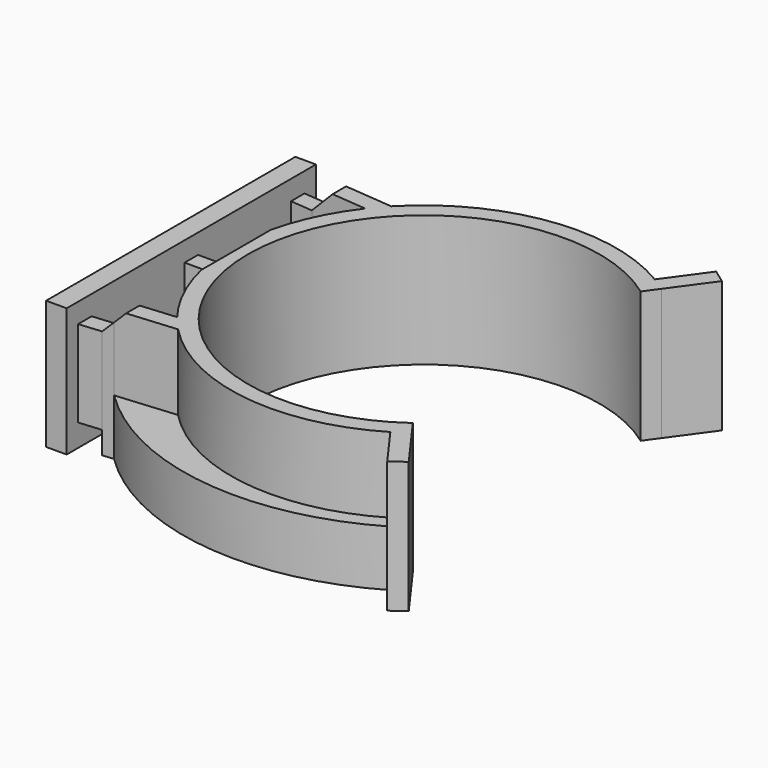
from build123d import *

# Parameters (mm, degrees)
F1_DEPTH = 11.74
F2_DEPTH = 5
F3_START = 2
F0_W     = 2
F0_H     = 1.5
F3_DEPTH = 7.74
F4_START = 2
F4_DEPTH = 3
F5_SIZE  = 2
F6_DEPTH = 11.5


# Not quite as in the source:
# - a feature names something its author has since deleted; it is built from what else it names


with BuildPart() as f1:
    # F0 (on Top) → F1 (new body)
    with BuildSketch(Plane.XY):
        with BuildLine():
            Line((5.4135556037, 0.75), (3.84, 0.75))
            Line((3.84, 0.75), (3.84, -0.75))
            Line((3.84, -0.75), (5.4135556037, -0.75))
            ThreePointArc((5.4135556037, -0.75), (5.3971960795, 0), (5.4135556037, 0.75))
        make_face()
        with BuildLine():
            ThreePointArc((10.1768930953, 11.8985744432), (9.5563193063, 11.2149691478), (8.9733212638, 10.499049243))
            ThreePointArc((8.9733212638, 10.499049243), (6.4405646269, 5.8994287949), (5.4135556037, 0.75))
            ThreePointArc((5.4135556037, 0.75), (5.3971960795, 0), (5.4135556037, -0.75))
            ThreePointArc((5.4135556037, -0.75), (6.4405646269, -5.8994287949), (8.9733212638, -10.499049243))
            ThreePointArc((8.9733212638, -10.499049243), (9.5563193063, -11.2149691478), (10.1768930953, -11.8985744432))
            ThreePointArc((10.1768930953, -11.8985744432), (20.3005620248, -17.0459811105), (31.425549646, -14.7614421147))
            ThreePointArc((31.425549646, -14.7614421147), (32.0614181574, -14.3620507052), (32.6792487822, -13.9352866242))
            Line((32.6792487822, -13.9352866242), (31.8, -12.72))
            ThreePointArc((31.8, -12.72), (6.8971960795, 0), (31.8, 12.72))
            Line((31.8, 12.72), (32.6792487822, 13.9352866242))
            ThreePointArc((32.6792487822, 13.9352866242), (32.0614181574, 14.3620507052), (31.425549646, 14.7614421147))
            ThreePointArc((31.425549646, 14.7614421147), (20.3005620248, 17.0459811105), (10.1768930953, 11.8985744432))
        make_face()
        with BuildLine():
            Line((31.425549646, -14.7614421147), (32.2020357723, -15.8346914866))
            Line((32.2020357723, -15.8346914866), (34.0313686021, -18.3631723491))
            Line((34.0313686021, -18.3631723491), (35.2466552263, -17.4839235669))
            Line((35.2466552263, -17.4839235669), (32.6792487822, -13.9352866242))
            ThreePointArc((32.6792487822, -13.9352866242), (32.0614181574, -14.3620507052), (31.425549646, -14.7614421147))
        make_face()
        with BuildLine():
            Line((34.0313686021, 18.3631723491), (32.2020357723, 15.8346914866))
            Line((32.2020357723, 15.8346914866), (31.425549646, 14.7614421147))
            ThreePointArc((31.425549646, 14.7614421147), (32.0614181574, 14.3620507052), (32.6792487822, 13.9352866242))
            Line((32.6792487822, 13.9352866242), (35.2466552263, 17.4839235669))
            Line((35.2466552263, 17.4839235669), (34.0313686021, 18.3631723491))
        make_face()
        with BuildLine():
            Line((4.84, 12.37), (3.84, 12.4583333333))
            Line((3.84, 12.4583333333), (3.84, 10.9524926213))
            Line((3.84, 10.9524926213), (8.9733212638, 10.499049243))
            ThreePointArc((8.9733212638, 10.499049243), (9.5563193063, 11.2149691478), (10.1768930953, 11.8985744432))
            Line((10.1768930953, 11.8985744432), (4.84, 12.37))
        make_face()
        with BuildLine():
            Line((3.84, -10.9524926213), (3.84, -12.4583333333))
            Line((3.84, -12.4583333333), (4.84, -12.37))
            Line((4.84, -12.37), (10.1768930953, -11.8985744432))
            ThreePointArc((10.1768930953, -11.8985744432), (9.5563193063, -11.2149691478), (8.9733212638, -10.499049243))
            Line((8.9733212638, -10.499049243), (3.84, -10.9524926213))
        make_face()
    extrude(amount=F1_DEPTH)

    # F0 (on Top) → F2 (join)
    with BuildSketch(Plane.XY):
        with BuildLine():
            ThreePointArc((32.2020357723, 15.8346914866), (17.9343865068, 18.7352052196), (4.84, 12.37))
            Line((4.84, 12.37), (10.1768930953, 11.8985744432))
            ThreePointArc((10.1768930953, 11.8985744432), (20.3005620248, 17.0459811105), (31.425549646, 14.7614421147))
            Line((31.425549646, 14.7614421147), (32.2020357723, 15.8346914866))
        make_face()
        with BuildLine():
            Line((10.1768930953, -11.8985744432), (4.84, -12.37))
            ThreePointArc((4.84, -12.37), (17.9343865068, -18.7352052196), (32.2020357723, -15.8346914866))
            Line((32.2020357723, -15.8346914866), (31.425549646, -14.7614421147))
            ThreePointArc((31.425549646, -14.7614421147), (20.3005620248, -17.0459811105), (10.1768930953, -11.8985744432))
        make_face()
        with BuildLine():
            Line((3.84, -0.75), (3.84, -10.9524926213))
            Line((3.84, -10.9524926213), (8.9733212638, -10.499049243))
            ThreePointArc((8.9733212638, -10.499049243), (6.4405646269, -5.8994287949), (5.4135556037, -0.75))
            Line((5.4135556037, -0.75), (3.84, -0.75))
        make_face()
        with BuildLine():
            Line((8.9733212638, 10.499049243), (3.84, 10.9524926213))
            Line((3.84, 10.9524926213), (3.84, 0.75))
            Line((3.84, 0.75), (5.4135556037, 0.75))
            ThreePointArc((5.4135556037, 0.75), (6.4405646269, 5.8994287949), (8.9733212638, 10.499049243))
        make_face()
    extrude(amount=F2_DEPTH)

    # F5
    f5_edges = [f1.edges().sort_by_distance(p)[0] for p in [
        (3.84, 0, 11.74),
        (3.84, -11.705413, 11.74),
        (3.84, 11.705413, 11.74),
    ]]
    chamfer(f5_edges, length=F5_SIZE)


with BuildPart() as f3:
    # F0 (on Top) → F3 (new body)
    with BuildSketch(Plane.XY.offset(F3_START)):
        with Locations((2.84, 0)):
            Rectangle(F0_W, F0_H)
    extrude(amount=F3_DEPTH)


with BuildPart() as f3b:
    # F0 (on Top) → F3, piece 2 (new body)
    with BuildSketch(Plane.XY.offset(F3_START)):
        Polygon((1.84, -11.129159288), (1.84, -12.635), (3.84, -12.4583333333), (3.84, -10.9524926213), align=None)
    extrude(amount=F3_DEPTH)


with BuildPart() as f3c:
    # F0 (on Top) → F3, piece 3 (new body)
    with BuildSketch(Plane.XY.offset(F3_START)):
        Polygon((3.84, 12.4583333333), (1.84, 12.635), (1.84, 11.129159288), (3.84, 10.9524926213), align=None)
    extrude(amount=F3_DEPTH)


with BuildPart() as f4:
    # F0 (on Top) → F4 (new body)
    with BuildSketch(Plane.XY.offset(F4_START)):
        Polygon((3.84, 10.9524926213), (1.84, 11.129159288), (1.84, 0.75), (3.84, 0.75), align=None)
    extrude(amount=F4_DEPTH)


with BuildPart() as f4b:
    # F0 (on Top) → F4, piece 2 (new body)
    with BuildSketch(Plane.XY.offset(F4_START)):
        Polygon((1.84, -0.75), (1.84, -11.129159288), (3.84, -10.9524926213), (3.84, -0.75), align=None)
    extrude(amount=F4_DEPTH)


with BuildPart() as f6:
    # F0 (on Top) → F6 (new body)
    with BuildSketch(Plane.XY):
        Polygon((1.84, 13.915), (0, 13.915), (0, -13.915), (1.84, -13.915), (1.84, -12.635), (1.84, -11.129159288), (1.84, -0.75), (1.84, 0.75), (1.84, 11.129159288), (1.84, 12.635), align=None)
    extrude(amount=F6_DEPTH)


solid = Compound([f1.part, f3.part, f3b.part, f3c.part, f4.part, f4b.part, f6.part])
